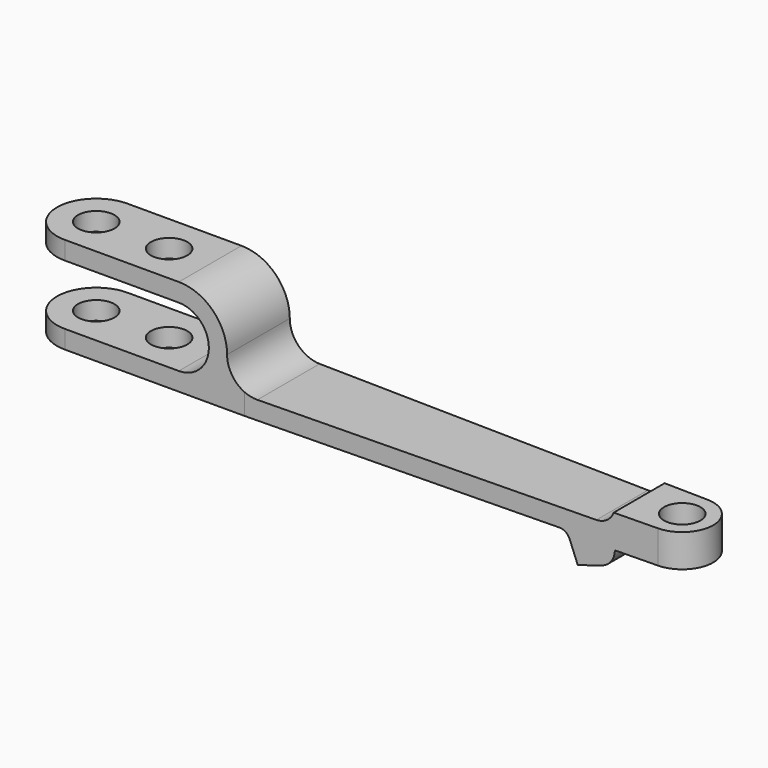
from build123d import *

# Parameters (mm, degrees)
F1_DEPTH = 1.075
F2_W     = 20.9250352345
F2_H     = 5.8195129968
F2_R     = 0.5
F3_DEPTH = 12.5
F4_R     = 0.5
F5_DEPTH = 12.5


# Not quite as in the source:
# - ends of sketch curves that miss each other by under 0.0002 mm in the source are joined


with BuildPart() as f1:
    # F0 (on Front) → F1 (new body, symmetric)
    with BuildSketch(Plane.XZ):
        with BuildLine():
            Line((0, 0.5), (0, 0))
            Line((0, 0), (14.5, 0))
            ThreePointArc((14.5, 0), (14.6687831398, -0.051983364), (14.7790735103, -0.1899183219))
            Line((14.7790735103, -0.1899183219), (15, -0.75))
            Line((15, -0.75), (15.645704163, -0.55329938))
            ThreePointArc((15.645704163, -0.55329938), (15.8994973246, -0.3756690667), (15.9999418448, -0.082625733))
            Line((15.9999418448, -0.082625733), (16, -0.075))
            Line((16, -0.075), (18, -0.075))
            Line((18, -0.075), (18, 0.825))
            Line((18, 0.825), (15.9683748499, 0.825))
            ThreePointArc((15.9683748499, 0.825), (15.7850438563, 0.5892080819), (15.5, 0.5))
            Line((15.5, 0.5), (6.35, 0.5))
            ThreePointArc((6.35, 0.5), (5.7666369055, 0.7416369055), (5.525, 1.325))
            ThreePointArc((5.525, 1.325), (5.4508825364, 1.7619415066), (5.2368220677, 2.15))
            Line((5.2368220677, 2.15), (4.2, 2.15))
            ThreePointArc((4.2, 2.15), (5.025, 1.325), (4.2, 0.5))
            Line((4.2, 0.5), (0, 0.5))
        make_face()
        with BuildLine():
            Line((0, 2.15), (4.2, 2.15))
            Line((4.2, 2.15), (5.2368220677, 2.15))
            ThreePointArc((5.2368220677, 2.15), (4.7755432217, 2.5184718262), (4.2, 2.65))
            Line((4.2, 2.65), (0, 2.65))
            Line((0, 2.65), (0, 2.15))
        make_face()
    extrude(amount=F1_DEPTH, both=True)

    # F2 (on Top) → F3 (cut, symmetric)
    with BuildSketch(Plane.XY):
        with Locations((8.4883153904, -0.0547866803)):
            Rectangle(F2_W, F2_H)
        with BuildLine():
            Line((6, 1.075), (17.1671358116, 0.8498272554))
            ThreePointArc((17.1671358116, 0.8498272554), (17.7570689581, 0.5949514939), (18, 0))
            ThreePointArc((18, 0), (17.7570689581, -0.5949514939), (17.1671358116, -0.8498272554))
            Line((17.1671358116, -0.8498272554), (6, -1.075))
            Line((6, -1.075), (1.075, -1.075))
            ThreePointArc((1.075, -1.075), (0.3148602102, -0.7601397898), (0, 0))
            ThreePointArc((0, 0), (0.3148602102, 0.7601397898), (1.075, 1.075))
            Line((1.075, 1.075), (6, 1.075))
        make_face(mode=Mode.SUBTRACT)
        with Locations((1.075, 0)):
            Circle(F2_R)
        with Locations((3.075, 0)):
            Circle(F2_R)
    extrude(amount=F3_DEPTH, both=True, mode=Mode.SUBTRACT)

    # F4 (on Top) → F5 (cut, symmetric)
    with BuildSketch(Plane.XY):
        with Locations((17.15, 0)):
            Circle(F4_R)
    extrude(amount=F5_DEPTH, both=True, mode=Mode.SUBTRACT)


solid = f1.part
